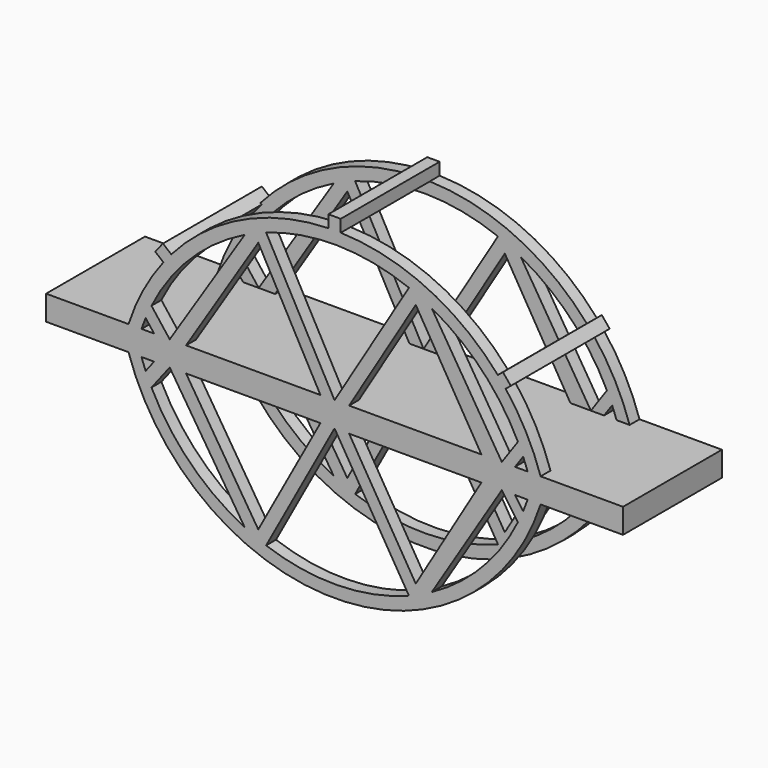
from build123d import *

# Parameters (mm, degrees)
F1_DEPTH  = 19.05
F2_DEPTH  = 3.81
F6_DEPTH  = 25.4
F8_DEPTH  = 25.4
F10_W     = 3.81
F10_H     = 38.1
F11_DEPTH = 1.905
F13_W     = 38.1
F13_H     = 3.81
F14_DEPTH = 1.905
F16_W     = 3.81
F16_H     = 38.1
F17_DEPTH = 1.905


with BuildPart() as f1:
    # F0 (on Front) → F1 (new body)
    with BuildSketch(Plane.XZ):
        Polygon((-46.9931786472, -25.5670996868), (-44.2826177091, -25.5670996868), (-11.655836644, -25.5670996868), (-6.0116577152, -25.5670996868), (12.9834232079, -25.5670996868), (19.9568117138, -25.5670996868), (39.0253004208, -25.5670996868), (44.6606800013, -25.5670996868), (77.2853784402, -25.5670996868), (80.0068213528, -25.5670996868), (80.0068213528, -21.7570996868), (75.986402619, -21.7570996868), (72.1197685419, -21.7570996868), (68.0612294563, -21.7570996868), (61.768413665, -21.7570996868), (20.9944943702, -21.7570996868), (16.5068213528, -21.7570996868), (12.1509924185, -21.7570996868), (-29.2575259188, -21.7570996868), (-34.2931786472, -21.7570996868), (-39.1061258363, -21.7570996868), (-42.9727599134, -21.7570996868), (-46.9931786472, -21.7570996868), align=None)
    extrude(amount=F1_DEPTH)

    # F0 (on Front) → F2 (join)
    with BuildSketch(Plane.XZ):
        with BuildLine():
            ThreePointArc((80.0068213528, -21.7570996868), (16.5068213528, 24.3272683475), (-46.9931786472, -21.7570996868))
            Line((-46.9931786472, -21.7570996868), (-42.9727599134, -21.7570996868))
            ThreePointArc((-42.9727599134, -21.7570996868), (-42.3584074876, -20.0701863071), (-41.6962231514, -18.4014689678))
            Line((-41.6962231514, -18.4014689678), (-39.1061258363, -21.7570996868))
            Line((-39.1061258363, -21.7570996868), (-34.2931786472, -21.7570996868))
            Line((-34.2931786472, -21.7570996868), (-29.2575259188, -21.7570996868))
            Line((-29.2575259188, -21.7570996868), (-7.0000388811, 13.3305896838))
            Line((-7.0000388811, 13.3305896838), (12.1509924185, -21.7570996868))
            Line((12.1509924185, -21.7570996868), (16.5068213528, -21.7570996868))
            Line((16.5068213528, -21.7570996868), (20.9944943702, -21.7570996868))
            Line((20.9944943702, -21.7570996868), (41.5369324101, 12.2571850479))
            Line((41.5369324101, 12.2571850479), (61.768413665, -21.7570996868))
            Line((61.768413665, -21.7570996868), (68.0612294563, -21.7570996868))
            Line((68.0612294563, -21.7570996868), (72.1197685419, -21.7570996868))
            Line((72.1197685419, -21.7570996868), (74.6210757351, -18.1878090206))
            ThreePointArc((74.6210757351, -18.1878090206), (75.3308173459, -19.9620963987), (75.986402619, -21.7570996868))
            Line((75.986402619, -21.7570996868), (80.0068213528, -21.7570996868))
        make_face()
        with BuildLine():
            Line((-11.178777875, 14.105789702), (-34.2931786472, -21.7570996868))
            Line((-34.2931786472, -21.7570996868), (-39.9135117304, -14.475611754))
            ThreePointArc((-39.9135117304, -14.475611754), (-27.9079970052, 2.18961195), (-11.178777875, 14.105789702))
        make_face(mode=Mode.SUBTRACT)
        with BuildLine():
            Line((39.429121883, 16.1977747781), (16.5068213528, -21.7570996868))
            Line((16.5068213528, -21.7570996868), (-4.5823001378, 16.8814745176))
            ThreePointArc((-4.5823001378, 16.8814745176), (17.3205828823, 20.512010904), (39.1223416395, 16.3167285364))
            ThreePointArc((39.1223416395, 16.3167285364), (39.2758094437, 16.2574519995), (39.429121883, 16.1977747781))
        make_face(mode=Mode.SUBTRACT)
        with BuildLine():
            Line((73.0250629731, -14.6738574973), (68.0612294563, -21.7570996868))
            Line((68.0612294563, -21.7570996868), (46.4705336291, 12.932825192))
            ThreePointArc((46.4705336291, 12.932825192), (61.8975067378, 1.1972620156), (73.0250629731, -14.6738574973))
        make_face(mode=Mode.SUBTRACT)
        Polygon((-46.9931786472, -25.5670996868), (-44.2826177091, -25.5670996868), (-11.655836644, -25.5670996868), (-6.0116577152, -25.5670996868), (12.9834232079, -25.5670996868), (19.9568117138, -25.5670996868), (39.0253004208, -25.5670996868), (44.6606800013, -25.5670996868), (77.2853784402, -25.5670996868), (80.0068213528, -25.5670996868), (80.0068213528, -21.7570996868), (75.986402619, -21.7570996868), (72.1197685419, -21.7570996868), (68.0612294563, -21.7570996868), (61.768413665, -21.7570996868), (20.9944943702, -21.7570996868), (16.5068213528, -21.7570996868), (12.1509924185, -21.7570996868), (-29.2575259188, -21.7570996868), (-34.2931786472, -21.7570996868), (-39.1061258363, -21.7570996868), (-42.9727599134, -21.7570996868), (-46.9931786472, -21.7570996868), align=None)
    extrude(amount=F2_DEPTH)

    # F3: F1 across face


with BuildPart() as f1_1:
    add(f1.part)
    add(f1.part.mirror(Plane(origin=(16.5068213528, -19.05, -23.6620996868), x_dir=(1, 0, 0), z_dir=(0, -1, 0))))

    # F4: F1 across face


with BuildPart() as f1_2:
    add(f1_1.part)
    add(f1_1.part.mirror(Plane(origin=(16.5068213528, -19.05, -25.5670996868), x_dir=(1, 0, 0), z_dir=(0, 0, -1))))

    # F5 (on face) → F6 (join)
    with BuildSketch(Plane.YZ.offset(80.0068213528)):
        Polygon((-34.29, -21.7570996868), (-38.1, -21.7570996868), (-38.1, -29.3770996868), (-34.29, -29.3770996868), (-3.81, -29.3770996868), (0, -29.3770996868), (0, -21.7570996868), (-3.81, -21.7570996868), align=None)
    extrude(amount=F6_DEPTH)

    # F7 (on face) → F8 (join)
    with BuildSketch(Plane(origin=(-46.9931786472, 0, 0), x_dir=(0, -1, 0), z_dir=(-1, 0, 0))):
        Polygon((3.81, -21.7570996868), (0, -21.7570996868), (0, -29.3770996868), (3.81, -29.3770996868), (34.29, -29.3770996868), (38.1, -29.3770996868), (38.1, -21.7570996868), (34.29, -21.7570996868), align=None)
    extrude(amount=F8_DEPTH)

    # F10 (on line) → F11 (join, symmetric)
    with BuildSketch(Plane(origin=(27.5104913128, 0, -33.4001606198), x_dir=(0.7718794649, 0, 0.6357688981), z_dir=(-0.6357688981, 0, 0.7718794649))):
        with Locations((52.6225773382, -19.05)):
            Rectangle(F10_W, F10_H)
    extrude(amount=F11_DEPTH, both=True)

    # F13 (on line) → F14 (join, symmetric)
    with BuildSketch(Plane(origin=(16.5068213528, 0, 0), x_dir=(0, -1, 0), z_dir=(-1, 0, 0))):
        with Locations((19.05, 26.1732695389)):
            Rectangle(F13_W, F13_H)
    extrude(amount=F14_DEPTH, both=True)

    # F16 (on line) → F17 (join, symmetric)
    with BuildSketch(Plane(origin=(-14.1663078752, 0, -17.1991460654), x_dir=(0.7718794649, 0, -0.6357688981), z_dir=(-0.6357688981, 0, -0.7718794649))):
        with Locations((-28.4333097053, 19.05)):
            Rectangle(F16_W, F16_H)
    extrude(amount=F17_DEPTH, both=True)


solid = f1_2.part
